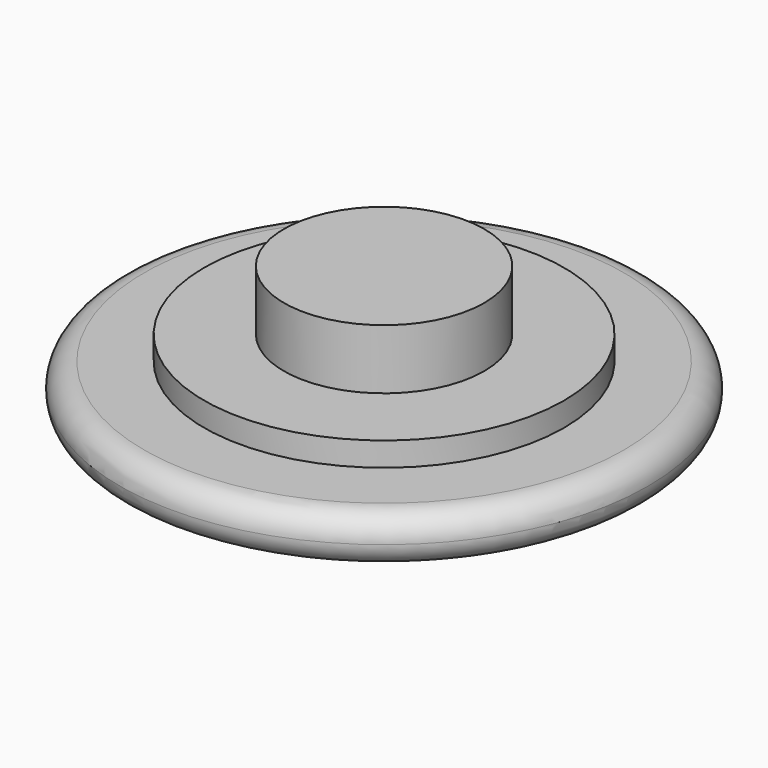
from build123d import *

# Parameters (mm, degrees)
F0_R         = 11
F0_R_2       = 7.5
F1_DEPTH     = 2
F0_R_3       = 4.175
F2_DEPTH     = 3
F3_DEPTH     = 5.5
F4_R         = 0.99999
F5_TEXT_SIZE = 5.2867677398
F6_DEPTH     = 1


# Not quite as in the source:
# - a fillet or chamfer is up to 0.001 mm smaller than in the source, because OpenCascade refuses the exact size
# - Text() gives the source's letters only with a copy of the font that has no kerning and outlines rounded to 1/6400 em; it was checked with that copy


with BuildPart() as f1:
    # F0 (on Top) → F1 (new body)
    with BuildSketch(Plane.XY):
        Circle(F0_R)
        Circle(F0_R_2, mode=Mode.SUBTRACT)
    extrude(amount=F1_DEPTH)

    # F0 (on Top) → F2 (join)
    with BuildSketch(Plane.XY):
        Circle(F0_R_2)
        Circle(F0_R_3, mode=Mode.SUBTRACT)
    extrude(amount=F2_DEPTH)

    # F0 (on Top) → F3 (join)
    with BuildSketch(Plane.XY):
        Circle(F0_R_3)
    extrude(amount=F3_DEPTH)

    # F4 (radius 1 in the source; OpenCascade refuses exactly that, so slightly less here)
    f4_edges = [f1.edges().sort_by_distance(p)[0] for p in [
        (-11, 0, 2),
        (-11, 0, 0),
    ]]
    fillet(f4_edges, radius=F4_R)

    # F5 (on face) → F6 (cut)
    with BuildSketch(Plane(origin=(0, 0, 0), x_dir=(1, 0, 0), z_dir=(0, 0, -1))):
        with Locations((-9.8325809795, -1.8221831086)):
            Text('Breathe', F5_TEXT_SIZE, font='Open Sans', text_align=(TextAlign.LEFT, TextAlign.BOTTOM))
    extrude(amount=-F6_DEPTH, mode=Mode.SUBTRACT)


solid = f1.part
